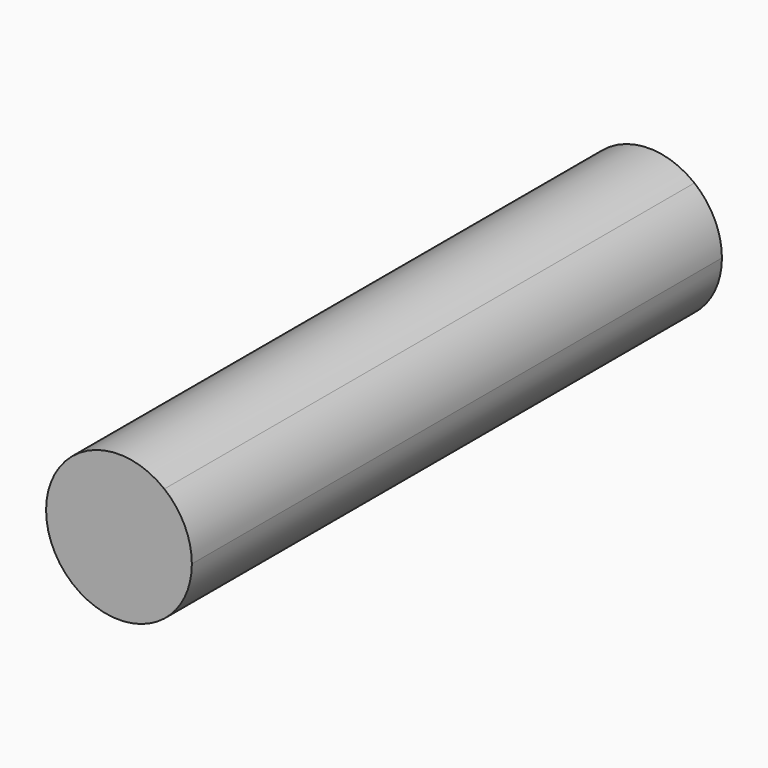
from build123d import *

# Parameters (mm, degrees)
F1_DEPTH = 50


# Not quite as in the source:
# - a feature of the source that left no trace in its solid (it failed there, or was rolled back) is left out


with BuildPart() as f1:
    # F0 (on Front) → F1 (new body, symmetric)
    with BuildSketch(Plane.XZ):
        with BuildLine():
            ThreePointArc((-7.2535058055, -8.6087479297), (-4.1934333127, -4.7789399387), (-3.101093635, 0))
            ThreePointArc((-3.101093635, 0), (-4.1934333127, 4.7789399387), (-7.2535058055, 8.6087479297))
            ThreePointArc((-7.2535058055, 8.6087479297), (-25.101093635, 0), (-7.2535058055, -8.6087479297))
        make_face()
    extrude(amount=F1_DEPTH, both=True)


solid = f1.part
